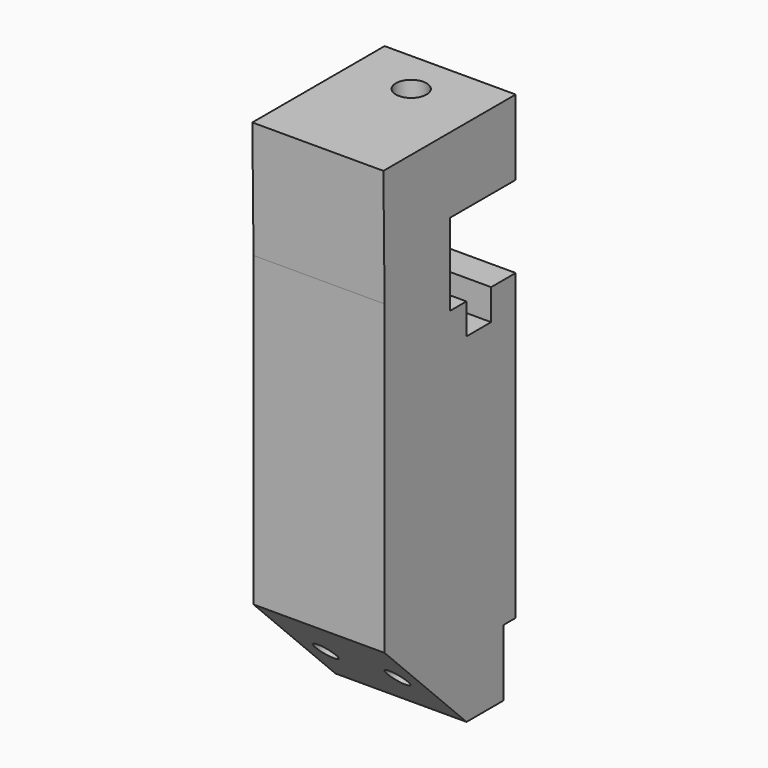
from build123d import *

# Parameters (mm, degrees)
F0_W      = 5.55
F0_H      = 2.45
F1_DEPTH  = 6.4
F3_DEPTH  = 9.3
F2_R      = 1.5
F4_DEPTH  = 11.8
F5_DEPTH  = 3
F6_SIZE   = 10
F9_DEPTH  = 10
F10_R     = 1
F11_DEPTH = 16.7
F13_SIZE  = 3
F12_R     = 3.1718540483
F12_R_2   = 3.2332055741
F14_DEPTH = 11.3
F15_SIZE2 = 9.99999
F15_SIZE  = 4.99999


# Not quite as in the source:
# - a fillet or chamfer is up to 0.001 mm smaller than in the source, because OpenCascade refuses the exact size
# - a feature names something its author has since deleted; it is built from what else it names


with BuildPart() as f1:
    # F0 (on Right) → F1 (new body, symmetric)
    with BuildSketch(Plane.YZ):
        Polygon((-8, -3.8421934836), (-8, 0), (-16, 0), (-16, -40), (-1.5, -40), (-1.5, -33.5), (0, -33.5), (0, -3.8421934836), (-3, -3.8421934836), (-3, -6.8521934836), (-6.01, -6.8521934836), (-6.01, -3.8421934836), align=None)
        Polygon((-8, 4.1578065164), (0, 4.1578065164), (0, 8.6438981816), (0, 11.5000782534), (-16.1481745615, 11.5000782534), (-16, 0), (-8, 0), align=None)
        with Locations((-4.2636177904, 7.6219322528)):
            Rectangle(F0_W, F0_H, mode=Mode.SUBTRACT)
        with Locations((-4.2636177904, 7.6219322528)):
            Rectangle(F0_W, F0_H)
    extrude(amount=F1_DEPTH, both=True)

    # F0 (on Right) → F3 (cut)
    with BuildSketch(Plane.YZ):
        with Locations((-4.2636177904, 7.6219322528)):
            Rectangle(F0_W, F0_H)
    extrude(amount=-F3_DEPTH, mode=Mode.SUBTRACT)

    # F2 (on face) → F4 (cut)
    with BuildSketch(Plane.XY.offset(11.5000782534)):
        with Locations((-0.4, -4.2524)):
            Circle(F2_R)
    extrude(amount=-F4_DEPTH, mode=Mode.SUBTRACT)

    # F0 (on Right) → F5 (cut)
    with BuildSketch(Plane.YZ):
        with Locations((-4.2636177904, 7.6219322528)):
            Rectangle(F0_W, F0_H)
    extrude(amount=F5_DEPTH, mode=Mode.SUBTRACT)

    # F6
    f6_edges = [f1.edges().sort_by_distance(p)[0] for p in [
        (0, -16, -40),
    ]]
    chamfer(f6_edges, length=F6_SIZE)

    # F7 (on face) → F9 (cut)
    with BuildSketch(Plane(origin=(-6.4, 0, 0), x_dir=(0, -1, 0), z_dir=(-1, 0, 0))):
        Polygon((3, -6.8521934836), (3, -4.8421934836), (1, -4.8421934836), (1, -14.3586024642), (1, -21.1353842169), (1, -32.5), (2.5, -32.5), (12.0857864376, -32.5), (15, -29.5857864376), (15, 0.006442061), (15.135206901, 10.5000782534), (7.8539028764, 10.5000782534), (7.8539028764, 5.1578065164), (9, 5.1578065164), (9, -4.8421934836), (6.01, -4.8421934836), (6.01, -6.8521934836), align=None)
    extrude(amount=-F9_DEPTH, mode=Mode.SUBTRACT)

    # F10 (on face) → F11 (cut)
    with BuildSketch(Plane(origin=(0, -1.5, 0), x_dir=(-1, 0, 0), z_dir=(0, 1, 0))):
        with Locations((-3.5, -35.2)):
            Circle(F10_R)
        with Locations((3.5, -35.2)):
            Circle(F10_R)
    extrude(amount=-F11_DEPTH, mode=Mode.SUBTRACT)

    # F13
    f13_edges = [f1.edges().sort_by_distance(p)[0] for p in [
        (3.6, -6.542893, -32.5),
        (-1.4, -1, -32.5),
    ]]
    chamfer(f13_edges, length=F13_SIZE)

    # F12 (on face) → F14 (cut)
    with BuildSketch(Plane(origin=(0, 0, 0), x_dir=(-1, 0, 0), z_dir=(0, 1, 0))):
        with Locations((0, -12.6159423962)):
            Circle(F12_R)
        with Locations((0, -27.5774579495)):
            Circle(F12_R_2)
    extrude(amount=-F14_DEPTH, mode=Mode.SUBTRACT)

    # F15 (size 5 and 10 in the source; OpenCascade refuses exactly that, so slightly less here)
    f15_edges = [f1.edges().sort_by_distance(p)[0] for p in [
        (3.6, -7.505, -4.842193),
        (3.6, -9, 0.157807),
        (3.6, -8.426951, 5.157807),
    ]]
    f15_side = f1.faces().sort_by_distance((3.6, -8.906235, -12.735974))[0]
    chamfer(f15_edges, length=F15_SIZE, length2=F15_SIZE2, reference=f15_side)


solid = f1.part
